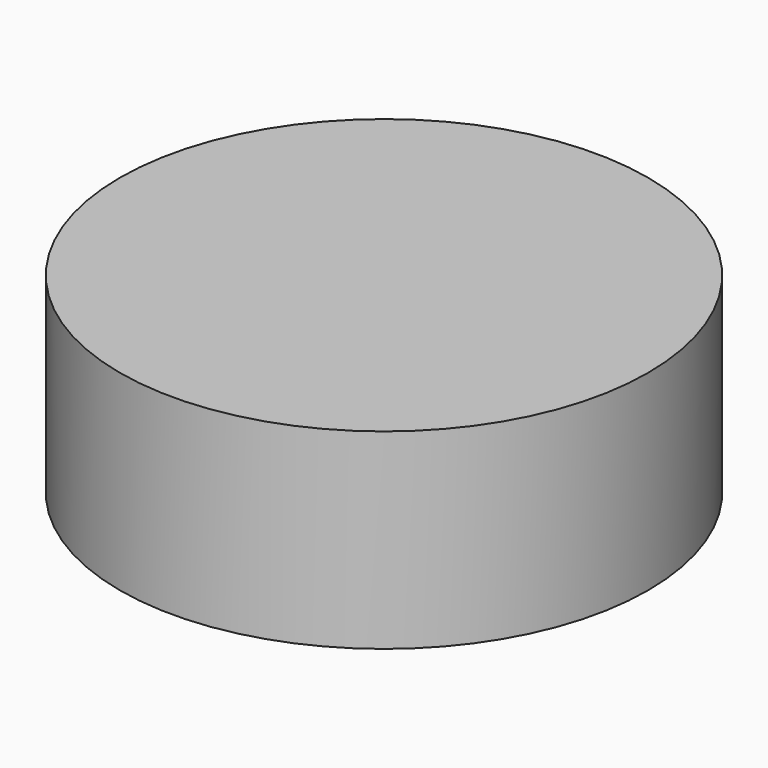
from build123d import *

# Parameters (mm, degrees)
F0_W = 47.9319319129
F0_H = 34.7506478429


# Not quite as in the source:
# - the program builds the solid bodies; features that only make, move or delete a surface that nothing else refers to are left out


with BuildPart() as f1:
    # F0 (on Front) → F1 (revolve)
    with BuildSketch(Plane.XZ):
        with Locations((-23.9659659564, 17.3753239214)):
            Rectangle(F0_W, F0_H)
    revolve(axis=Axis((0, 0, 17.3753239214), (0, 0, 1)))


solid = f1.part
